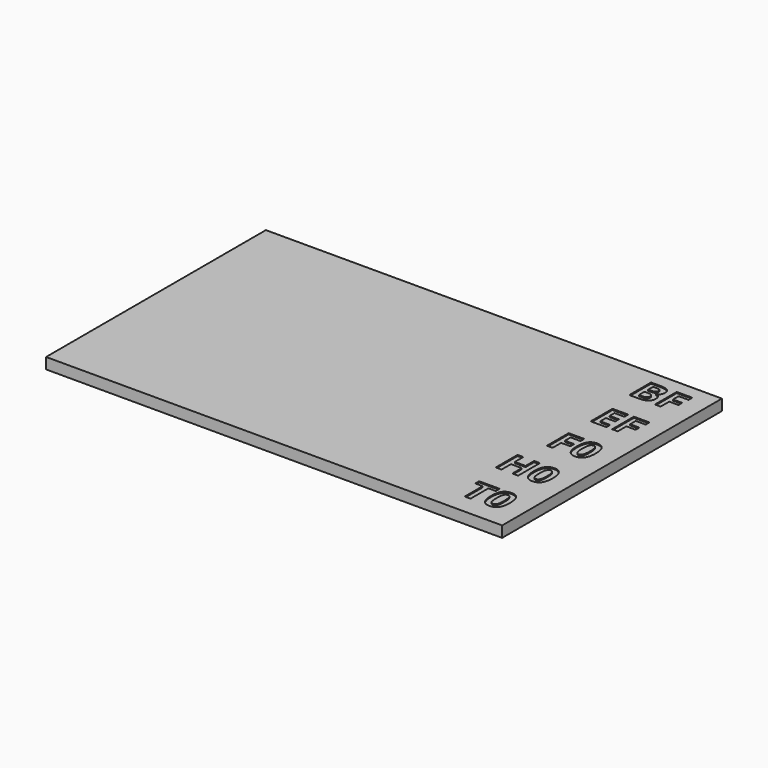
from build123d import *

# Parameters (mm, degrees)
F0_W         = 83
F0_H         = 50
F1_DEPTH     = 2
F2_TEXT_SIZE = 6.9444444444
F3_DEPTH     = 0.2


# Not quite as in the source:
# - Text() gives the source's letters only with a copy of the font that has no kerning and outlines rounded to 1/6400 em; it was checked with that copy


with BuildPart() as f1:
    # F0 (on Top) → F1 (new body)
    with BuildSketch(Plane.XY):
        with Locations((-41.5, 25)):
            Rectangle(F0_W, F0_H)
    extrude(amount=F1_DEPTH)

    # F2 (on face) → F3 (cut)
    with BuildSketch(Plane.XY.offset(2)):
        with Locations((-11.5818142361, 42.625)):
            Text('BF', F2_TEXT_SIZE, font='Open Sans', font_style=FontStyle.BOLD, text_align=(TextAlign.LEFT, TextAlign.BOTTOM))
        with Locations((-10.8049045139, 32.875)):
            Text('EF', F2_TEXT_SIZE, font='Open Sans', font_style=FontStyle.BOLD, text_align=(TextAlign.LEFT, TextAlign.BOTTOM))
        with Locations((-10.978515625, 23.125)):
            Text('F0', F2_TEXT_SIZE, font='Open Sans', font_style=FontStyle.BOLD, text_align=(TextAlign.LEFT, TextAlign.BOTTOM))
        with Locations((-12.4802517361, 13.375)):
            Text('H0', F2_TEXT_SIZE, font='Open Sans', font_style=FontStyle.BOLD, text_align=(TextAlign.LEFT, TextAlign.BOTTOM))
        with Locations((-11.1879340278, 3.625)):
            Text('T0', F2_TEXT_SIZE, font='Open Sans', font_style=FontStyle.BOLD, text_align=(TextAlign.LEFT, TextAlign.BOTTOM))
    extrude(amount=-F3_DEPTH, mode=Mode.SUBTRACT)


solid = f1.part
